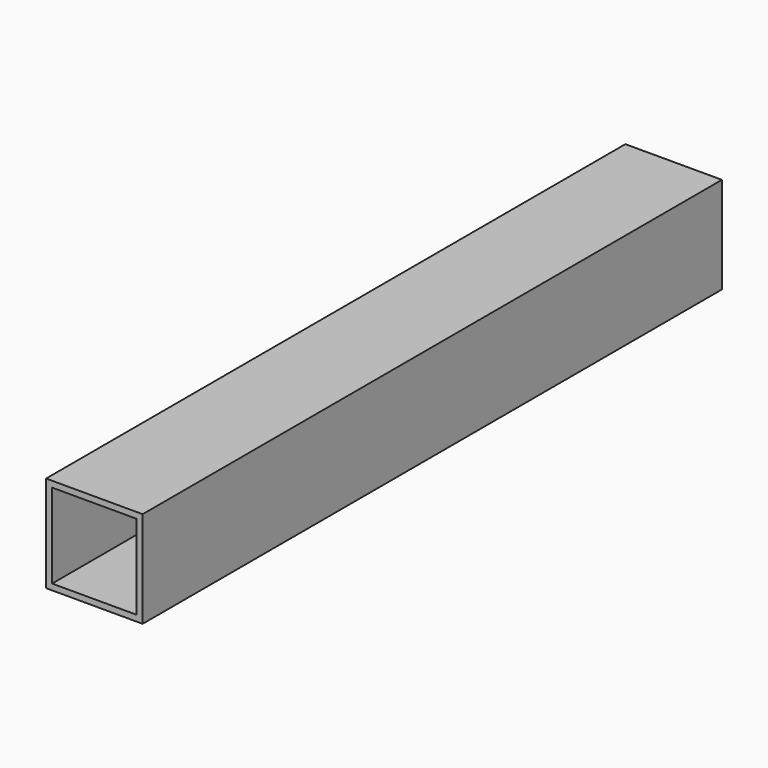
from build123d import *

# Parameters (mm, degrees)
F0_W     = 40
F0_H     = 40
F0_W_2   = 35
F0_H_2   = 35
F1_DEPTH = 300


# Not quite as in the source:
# - a feature names something its author has since deleted; it is built from what else it names


with BuildPart() as f1:
    # F0 (on Front) → F1 (new body)
    with BuildSketch(Plane.XZ):
        Rectangle(F0_W, F0_H)
        Rectangle(F0_W_2, F0_H_2, mode=Mode.SUBTRACT)
    extrude(amount=F1_DEPTH)


solid = f1.part
